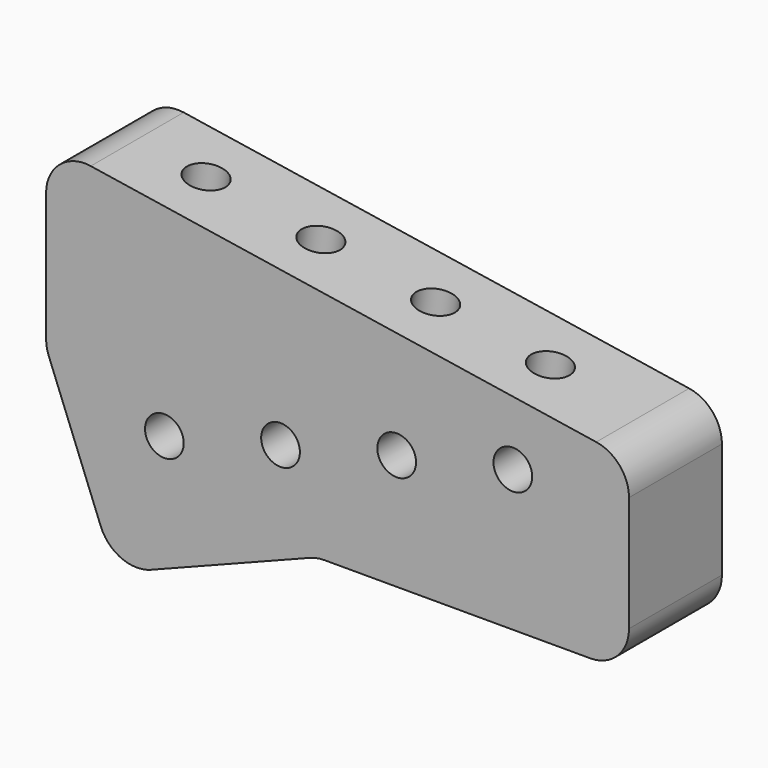
from build123d import *

# Parameters (mm, degrees)
F0_R     = 2.54
F1_DEPTH = 15.24
F2_R     = 5.08
F3_R     = 2.54
F4_DEPTH = 15.748


with BuildPart() as f1:
    # F0 (on Front) → F1 (new body)
    with BuildSketch(Plane.XZ):
        Polygon((-26.816706221, 12.8465024581), (-26.816706221, -10.6672204749), (-26.816706221, -10.8938248026), (-17.7876478214, -33.9755966375), (8.7138581745, -23.6088168675), (49.6632434885, -23.6088168675), (49.6632434885, 0.9602710623), align=None)
        with Locations((-11.2967565115, -16.1095818214)):
            Circle(F0_R, mode=Mode.SUBTRACT)
        with Locations((3.9432434885, -12.1794487806)):
            Circle(F0_R, mode=Mode.SUBTRACT)
        with Locations((19.1832434885, -8.4152225918)):
            Circle(F0_R, mode=Mode.SUBTRACT)
        with Locations((34.4232434885, -5.1024009119)):
            Circle(F0_R, mode=Mode.SUBTRACT)
    extrude(amount=F1_DEPTH)

    # F2
    f2_edges = [f1.edges().sort_by_distance(p)[0] for p in [
        (-26.816706, -7.62, 12.846502),
        (49.663243, -7.62, 0.960271),
        (49.663243, -7.62, -23.608817),
        (8.713858, -7.62, -23.608817),
        (-17.787648, -7.62, -33.975597),
        (-26.816706, -7.62, -10.893825),
    ]]
    fillet(f2_edges, radius=F2_R)

    # F3 (on face) → F4 (cut)
    with BuildSketch(Plane(origin=(1.3170078158, 0, 8.474064501), x_dir=(0.988137358, 0, -0.1535726597), z_dir=(0.1535726597, 0, 0.988137358))):
        with Locations((32.3229017764, -7.62)):
            Circle(F3_R)
        with Locations((17.0829017764, -7.62)):
            Circle(F3_R)
        with Locations((1.8429017764, -7.62)):
            Circle(F3_R)
        with Locations((-13.3970982236, -7.62)):
            Circle(F3_R)
    extrude(amount=-F4_DEPTH, mode=Mode.SUBTRACT)


solid = f1.part
